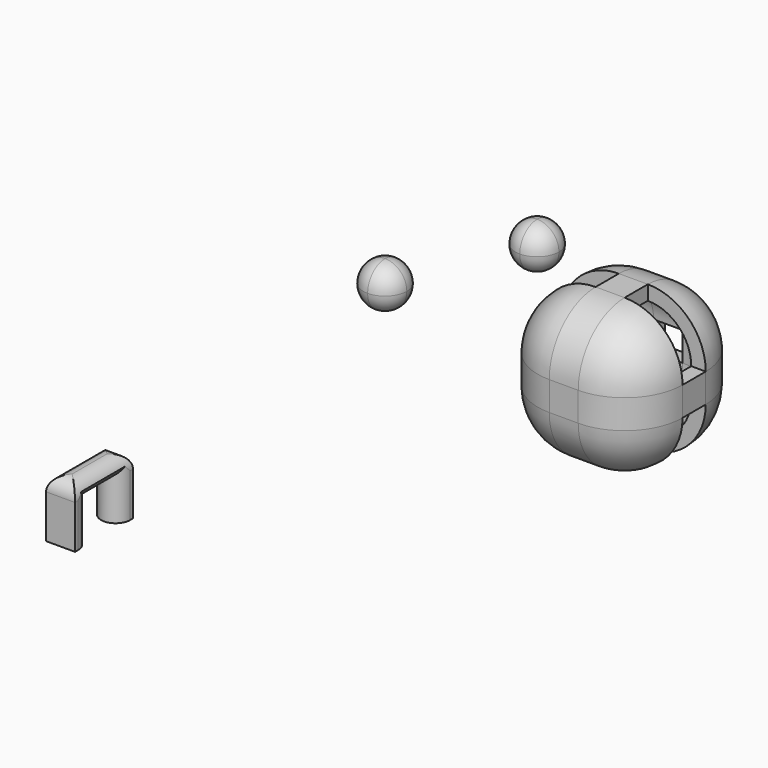
from build123d import *

# Parameters (mm, degrees)
F0_W         = 25.4
F0_H         = 25.4
F1_DEPTH     = 25.4
F2_R         = 10.16
F3_W         = 5.08
F3_H         = 12.7
F4_DEPTH     = 12.7
F6_DEPTH     = 5.08
F7_T1_DEPTH  = 5.08
F7_T3_DEPTH  = 6.35
F7_T5_DEPTH  = 9.525
F7_T7_DEPTH  = 12.7
F7_T13_DEPTH = 19.05
F7_T17_DEPTH = 11.43
F7_T24_DEPTH = 19.05
F7_T28_DEPTH = 11.43
F7_T35_DEPTH = 19.05
F7_T39_DEPTH = 11.43
F7_T46_DEPTH = 11.43
F7_T50_DEPTH = 19.05
F7_T57_DEPTH = 15.875
F7_T61_DEPTH = 12.7
F7_T68_DEPTH = 12.7
F7_T72_DEPTH = 15.875
F7_T79_DEPTH = 15.875
F7_T83_DEPTH = 12.7
F7_T90_DEPTH = 12.7
F7_T94_DEPTH = 15.875
F8_T         = 2.54
F9_W         = 7.62
F9_H         = 7.62
F10_DEPTH    = 7.62
F11_R        = 3.80999
F11_2_R      = 3.80999
F13_DEPTH    = 2.54
F15_DEPTH    = 2.54


# Not quite as in the source:
# - a fillet or chamfer that OpenCascade refuses, or shapes differently, is made with other operations: its cross-section is extruded or revolved along the edge and cut away or added
# - a fillet or chamfer is up to 0.001 mm smaller than in the source, because OpenCascade refuses the exact size
# - a shell that OpenCascade refuses in one call is made with other operations: the cavity is built on its own and cut out


with BuildPart() as f1:
    # F0 (on Top) → F1 (new body)
    with BuildSketch(Plane.XY):
        with Locations((-12.7, 12.7)):
            Rectangle(F0_W, F0_H)
    extrude(amount=F1_DEPTH)

    # F2
    f2_edges = [f1.edges().sort_by_distance(p)[0] for p in [
        (-12.7, 0, 25.4),
        (0, 12.7, 25.4),
        (-12.7, 25.4, 25.4),
        (-25.4, 12.7, 25.4),
        (-25.4, 0, 12.7),
        (0, 0, 12.7),
        (-12.7, 0, 0),
        (-25.4, 25.4, 12.7),
        (-25.4, 12.7, 0),
        (0, 25.4, 12.7),
        (-12.7, 25.4, 0),
        (0, 12.7, 0),
    ]]
    fillet(f2_edges, radius=F2_R)

    # F8: shell of thickness 2.54, made by hand


with BuildPart() as f4:
    # F3 (on Top) → F4 (new body)
    with BuildSketch(Plane.XY):
        with Locations((-51.7951508677, -55.0308073103)):
            Rectangle(F3_W, F3_H)
    extrude(amount=F4_DEPTH)

    # F5 (on face) → F6 (cut)
    with BuildSketch(Plane.YZ.offset(-49.2551508677)):
        Polygon((-58.2058073103, 0), (-55.0308073103, 0), (-51.8558073103, 0), (-51.8558073103, 9.525), (-58.2058073103, 9.525), align=None)
    extrude(amount=-F6_DEPTH, mode=Mode.SUBTRACT)

    # F7: fillet of radius 2.54 on 10 edges, made by hand

    # F7_s2 → F7_t1 (cut)
    with BuildSketch(Plane.YZ.offset(-54.3351508677)):
        with BuildLine():
            ThreePointArc((-51.2208073103, 12.7), (-49.4247560861, 11.9560512242), (-48.6808073103, 10.16))
            Line((-48.6808073103, 10.16), (-48.6300073103, 10.16))
            Line((-48.6300073103, 10.16), (-48.6300073103, 12.7508))
            Line((-48.6300073103, 12.7508), (-51.2208073103, 12.7508))
            Line((-51.2208073103, 12.7508), (-51.2208073103, 12.7))
        make_face()
        with BuildLine():
            ThreePointArc((-61.3808073103, 10.16), (-60.6368585346, 11.9560512242), (-58.8408073103, 12.7))
            Line((-58.8408073103, 12.7), (-58.8408073103, 12.7508))
            Line((-58.8408073103, 12.7508), (-61.4316073103, 12.7508))
            Line((-61.4316073103, 12.7508), (-61.4316073103, 10.16))
            Line((-61.4316073103, 10.16), (-61.3808073103, 10.16))
        make_face()
    extrude(amount=F7_T1_DEPTH, mode=Mode.SUBTRACT)

    # F7_s4 → F7_t3 (cut)
    with BuildSketch(Plane.XZ.offset(51.8558073103)):
        with BuildLine():
            ThreePointArc((-51.7951508677, 9.525), (-49.9990996435, 10.2689487758), (-49.2551508677, 12.065))
            Line((-49.2551508677, 12.065), (-49.2043508677, 12.065))
            Line((-49.2043508677, 12.065), (-49.2043508677, 9.4742))
            Line((-49.2043508677, 9.4742), (-51.7951508677, 9.4742))
            Line((-51.7951508677, 9.4742), (-51.7951508677, 9.525))
        make_face()
        with BuildLine():
            ThreePointArc((-54.3351508677, 12.065), (-53.5912020919, 10.2689487758), (-51.7951508677, 9.525))
            Line((-51.7951508677, 9.525), (-51.7951508677, 9.4742))
            Line((-51.7951508677, 9.4742), (-54.3859508677, 9.4742))
            Line((-54.3859508677, 9.4742), (-54.3859508677, 12.065))
            Line((-54.3859508677, 12.065), (-54.3351508677, 12.065))
        make_face()
    extrude(amount=F7_T3_DEPTH, mode=Mode.SUBTRACT)

    # F7_s6 → F7_t5 (cut)
    with BuildSketch(Plane.XY):
        with BuildLine():
            ThreePointArc((-51.7951508677, -58.2058073103), (-49.9990996435, -58.9497560861), (-49.2551508677, -60.7458073103))
            Line((-49.2551508677, -60.7458073103), (-49.2043508677, -60.7458073103))
            Line((-49.2043508677, -60.7458073103), (-49.2043508677, -58.1550073103))
            Line((-49.2043508677, -58.1550073103), (-51.7951508677, -58.1550073103))
            Line((-51.7951508677, -58.1550073103), (-51.7951508677, -58.2058073103))
        make_face()
        with BuildLine():
            ThreePointArc((-51.7951508677, -51.8558073103), (-49.9990996435, -51.1118585346), (-49.2551508677, -49.3158073103))
            Line((-49.2551508677, -49.3158073103), (-49.2043508677, -49.3158073103))
            Line((-49.2043508677, -49.3158073103), (-49.2043508677, -51.9066073103))
            Line((-49.2043508677, -51.9066073103), (-51.7951508677, -51.9066073103))
            Line((-51.7951508677, -51.9066073103), (-51.7951508677, -51.8558073103))
        make_face()
        with BuildLine():
            ThreePointArc((-54.3351508677, -49.3158073103), (-53.5912020919, -51.1118585346), (-51.7951508677, -51.8558073103))
            Line((-51.7951508677, -51.8558073103), (-51.7951508677, -51.9066073103))
            Line((-51.7951508677, -51.9066073103), (-54.3859508677, -51.9066073103))
            Line((-54.3859508677, -51.9066073103), (-54.3859508677, -49.3158073103))
            Line((-54.3859508677, -49.3158073103), (-54.3351508677, -49.3158073103))
        make_face()
        with BuildLine():
            ThreePointArc((-54.3351508677, -60.7458073103), (-53.5912020919, -58.9497560861), (-51.7951508677, -58.2058073103))
            Line((-51.7951508677, -58.2058073103), (-51.7951508677, -58.1550073103))
            Line((-51.7951508677, -58.1550073103), (-54.3859508677, -58.1550073103))
            Line((-54.3859508677, -58.1550073103), (-54.3859508677, -60.7458073103))
            Line((-54.3859508677, -60.7458073103), (-54.3351508677, -60.7458073103))
        make_face()
    extrude(amount=F7_T5_DEPTH, mode=Mode.SUBTRACT)

    # F7_s8 → F7_t7 (cut)
    with BuildSketch(Plane.XZ.offset(48.6808073103)):
        with BuildLine():
            ThreePointArc((-54.3351508677, 10.16), (-53.5912020919, 11.9560512242), (-51.7951508677, 12.7))
            Line((-51.7951508677, 12.7), (-51.7951508677, 12.7508))
            Line((-51.7951508677, 12.7508), (-54.3859508677, 12.7508))
            Line((-54.3859508677, 12.7508), (-54.3859508677, 10.16))
            Line((-54.3859508677, 10.16), (-54.3351508677, 10.16))
        make_face()
        with BuildLine():
            ThreePointArc((-51.7951508677, 12.7), (-49.9990996435, 11.9560512242), (-49.2551508677, 10.16))
            Line((-49.2551508677, 10.16), (-49.2043508677, 10.16))
            Line((-49.2043508677, 10.16), (-49.2043508677, 12.7508))
            Line((-49.2043508677, 12.7508), (-51.7951508677, 12.7508))
            Line((-51.7951508677, 12.7508), (-51.7951508677, 12.7))
        make_face()
    extrude(amount=F7_T7_DEPTH, mode=Mode.SUBTRACT)


with BuildPart() as f7_tool11:
    # F7_s12 → F7_t13 (new body)
    with BuildSketch(Plane.XZ.offset(61.3808073103)):
        with BuildLine():
            ThreePointArc((-51.7951508677, 12.7), (-49.9990996435, 11.9560512242), (-49.2551508677, 10.16))
            Line((-49.2551508677, 10.16), (-49.2043508677, 10.16))
            Line((-49.2043508677, 10.16), (-49.2043508677, 12.7508))
            Line((-49.2043508677, 12.7508), (-51.7951508677, 12.7508))
            Line((-51.7951508677, 12.7508), (-51.7951508677, 12.7))
        make_face()
    extrude(amount=-F7_T13_DEPTH)

    split(bisect_by=Plane.XZ.offset(48.6808073103), keep=Keep.BOTTOM)


with BuildPart() as f7_tool15:
    # F7_s16 → F7_t17 (new body)
    with BuildSketch(Plane.YZ.offset(-42.9051508677)):
        with BuildLine():
            ThreePointArc((-51.2208073103, 12.7), (-49.4247560861, 11.9560512242), (-48.6808073103, 10.16))
            Line((-48.6808073103, 10.16), (-48.6300073103, 10.16))
            Line((-48.6300073103, 10.16), (-48.6300073103, 12.7508))
            Line((-48.6300073103, 12.7508), (-51.2208073103, 12.7508))
            Line((-51.2208073103, 12.7508), (-51.2208073103, 12.7))
        make_face()
    extrude(amount=-F7_T17_DEPTH)

    split(bisect_by=Plane.YZ.offset(-49.2551508677), keep=Keep.TOP)


with BuildPart() as f7_tool11_1:
    add(f7_tool11.part)

    # F7_t19: intersect F7_tool15
    add(f7_tool15.part, mode=Mode.INTERSECT)


with BuildPart() as f4_1:
    add(f4.part)

    # F7_t9: cut F7_tool11
    add(f7_tool11_1.part, mode=Mode.SUBTRACT)


with BuildPart() as f7_tool22:
    # F7_s23 → F7_t24 (new body)
    with BuildSketch(Plane.XZ.offset(42.3308073103)):
        with BuildLine():
            ThreePointArc((-54.3351508677, 10.16), (-53.5912020919, 11.9560512242), (-51.7951508677, 12.7))
            Line((-51.7951508677, 12.7), (-51.7951508677, 12.7508))
            Line((-51.7951508677, 12.7508), (-54.3859508677, 12.7508))
            Line((-54.3859508677, 12.7508), (-54.3859508677, 10.16))
            Line((-54.3859508677, 10.16), (-54.3351508677, 10.16))
        make_face()
    extrude(amount=F7_T24_DEPTH)

    split(bisect_by=Plane.XZ.offset(48.6808073103), keep=Keep.BOTTOM)


with BuildPart() as f7_tool26:
    # F7_s27 → F7_t28 (new body)
    with BuildSketch(Plane.YZ.offset(-49.2551508677)):
        with BuildLine():
            ThreePointArc((-51.2208073103, 12.7), (-49.4247560861, 11.9560512242), (-48.6808073103, 10.16))
            Line((-48.6808073103, 10.16), (-48.6300073103, 10.16))
            Line((-48.6300073103, 10.16), (-48.6300073103, 12.7508))
            Line((-48.6300073103, 12.7508), (-51.2208073103, 12.7508))
            Line((-51.2208073103, 12.7508), (-51.2208073103, 12.7))
        make_face()
    extrude(amount=-F7_T28_DEPTH)

    split(bisect_by=Plane.YZ.offset(-54.3351508677), keep=Keep.BOTTOM)


with BuildPart() as f7_tool22_1:
    add(f7_tool22.part)

    # F7_t30: intersect F7_tool26
    add(f7_tool26.part, mode=Mode.INTERSECT)


with BuildPart() as f4_2:
    add(f4_1.part)

    # F7_t20: cut F7_tool22
    add(f7_tool22_1.part, mode=Mode.SUBTRACT)


with BuildPart() as f7_tool33:
    # F7_s34 → F7_t35 (new body)
    with BuildSketch(Plane.XZ.offset(48.6808073103)):
        with BuildLine():
            ThreePointArc((-54.3351508677, 10.16), (-53.5912020919, 11.9560512242), (-51.7951508677, 12.7))
            Line((-51.7951508677, 12.7), (-51.7951508677, 12.7508))
            Line((-51.7951508677, 12.7508), (-54.3859508677, 12.7508))
            Line((-54.3859508677, 12.7508), (-54.3859508677, 10.16))
            Line((-54.3859508677, 10.16), (-54.3351508677, 10.16))
        make_face()
    extrude(amount=F7_T35_DEPTH)

    split(bisect_by=Plane.XZ.offset(61.3808073103), keep=Keep.TOP)


with BuildPart() as f7_tool37:
    # F7_s38 → F7_t39 (new body)
    with BuildSketch(Plane.YZ.offset(-60.6851508677)):
        with BuildLine():
            ThreePointArc((-61.3808073103, 10.16), (-60.6368585346, 11.9560512242), (-58.8408073103, 12.7))
            Line((-58.8408073103, 12.7), (-58.8408073103, 12.7508))
            Line((-58.8408073103, 12.7508), (-61.4316073103, 12.7508))
            Line((-61.4316073103, 12.7508), (-61.4316073103, 10.16))
            Line((-61.4316073103, 10.16), (-61.3808073103, 10.16))
        make_face()
    extrude(amount=F7_T39_DEPTH)

    split(bisect_by=Plane.YZ.offset(-54.3351508677), keep=Keep.BOTTOM)


with BuildPart() as f7_tool33_1:
    add(f7_tool33.part)

    # F7_t41: intersect F7_tool37
    add(f7_tool37.part, mode=Mode.INTERSECT)


with BuildPart() as f4_3:
    add(f4_2.part)

    # F7_t31: cut F7_tool33
    add(f7_tool33_1.part, mode=Mode.SUBTRACT)


with BuildPart() as f7_tool44:
    # F7_s45 → F7_t46 (new body)
    with BuildSketch(Plane.YZ.offset(-54.3351508677)):
        with BuildLine():
            ThreePointArc((-61.3808073103, 10.16), (-60.6368585346, 11.9560512242), (-58.8408073103, 12.7))
            Line((-58.8408073103, 12.7), (-58.8408073103, 12.7508))
            Line((-58.8408073103, 12.7508), (-61.4316073103, 12.7508))
            Line((-61.4316073103, 12.7508), (-61.4316073103, 10.16))
            Line((-61.4316073103, 10.16), (-61.3808073103, 10.16))
        make_face()
    extrude(amount=F7_T46_DEPTH)

    split(bisect_by=Plane.YZ.offset(-49.2551508677), keep=Keep.TOP)


with BuildPart() as f7_tool48:
    # F7_s49 → F7_t50 (new body)
    with BuildSketch(Plane.XZ.offset(67.7308073103)):
        with BuildLine():
            ThreePointArc((-51.7951508677, 12.7), (-49.9990996435, 11.9560512242), (-49.2551508677, 10.16))
            Line((-49.2551508677, 10.16), (-49.2043508677, 10.16))
            Line((-49.2043508677, 10.16), (-49.2043508677, 12.7508))
            Line((-49.2043508677, 12.7508), (-51.7951508677, 12.7508))
            Line((-51.7951508677, 12.7508), (-51.7951508677, 12.7))
        make_face()
    extrude(amount=-F7_T50_DEPTH)

    split(bisect_by=Plane.XZ.offset(61.3808073103), keep=Keep.TOP)


with BuildPart() as f7_tool44_1:
    add(f7_tool44.part)

    # F7_t52: intersect F7_tool48
    add(f7_tool48.part, mode=Mode.INTERSECT)


with BuildPart() as f4_4:
    add(f4_3.part)

    # F7_t42: cut F7_tool44
    add(f7_tool44_1.part, mode=Mode.SUBTRACT)


with BuildPart() as f7_tool55:
    # F7_s56 → F7_t57 (new body)
    with BuildSketch(Plane.XY):
        with BuildLine():
            ThreePointArc((-51.7951508677, -51.8558073103), (-49.9990996435, -51.1118585346), (-49.2551508677, -49.3158073103))
            Line((-49.2551508677, -49.3158073103), (-49.2043508677, -49.3158073103))
            Line((-49.2043508677, -49.3158073103), (-49.2043508677, -51.9066073103))
            Line((-49.2043508677, -51.9066073103), (-51.7951508677, -51.9066073103))
            Line((-51.7951508677, -51.9066073103), (-51.7951508677, -51.8558073103))
        make_face()
    extrude(amount=F7_T57_DEPTH)

    split(bisect_by=Plane.XY.offset(9.525), keep=Keep.TOP)


with BuildPart() as f7_tool59:
    # F7_s60 → F7_t61 (new body)
    with BuildSketch(Plane.XZ.offset(45.5058073103)):
        with BuildLine():
            ThreePointArc((-51.7951508677, 9.525), (-49.9990996435, 10.2689487758), (-49.2551508677, 12.065))
            Line((-49.2551508677, 12.065), (-49.2043508677, 12.065))
            Line((-49.2043508677, 12.065), (-49.2043508677, 9.4742))
            Line((-49.2043508677, 9.4742), (-51.7951508677, 9.4742))
            Line((-51.7951508677, 9.4742), (-51.7951508677, 9.525))
        make_face()
    extrude(amount=F7_T61_DEPTH)

    split(bisect_by=Plane.XZ.offset(51.8558073103), keep=Keep.BOTTOM)


with BuildPart() as f7_tool55_1:
    add(f7_tool55.part)

    # F7_t63: intersect F7_tool59
    add(f7_tool59.part, mode=Mode.INTERSECT)


with BuildPart() as f4_5:
    add(f4_4.part)

    # F7_t53: cut F7_tool55
    add(f7_tool55_1.part, mode=Mode.SUBTRACT)


with BuildPart() as f7_tool66:
    # F7_s67 → F7_t68 (new body)
    with BuildSketch(Plane.XZ.offset(51.8558073103)):
        with BuildLine():
            ThreePointArc((-51.7951508677, 9.525), (-49.9990996435, 10.2689487758), (-49.2551508677, 12.065))
            Line((-49.2551508677, 12.065), (-49.2043508677, 12.065))
            Line((-49.2043508677, 12.065), (-49.2043508677, 9.4742))
            Line((-49.2043508677, 9.4742), (-51.7951508677, 9.4742))
            Line((-51.7951508677, 9.4742), (-51.7951508677, 9.525))
        make_face()
    extrude(amount=F7_T68_DEPTH)

    split(bisect_by=Plane.XZ.offset(58.2058073103), keep=Keep.TOP)


with BuildPart() as f7_tool70:
    # F7_s71 → F7_t72 (new body)
    with BuildSketch(Plane.XY.offset(15.875)):
        with BuildLine():
            ThreePointArc((-51.7951508677, -58.2058073103), (-49.9990996435, -58.9497560861), (-49.2551508677, -60.7458073103))
            Line((-49.2551508677, -60.7458073103), (-49.2043508677, -60.7458073103))
            Line((-49.2043508677, -60.7458073103), (-49.2043508677, -58.1550073103))
            Line((-49.2043508677, -58.1550073103), (-51.7951508677, -58.1550073103))
            Line((-51.7951508677, -58.1550073103), (-51.7951508677, -58.2058073103))
        make_face()
    extrude(amount=-F7_T72_DEPTH)

    split(bisect_by=Plane.XY.offset(9.525), keep=Keep.TOP)


with BuildPart() as f7_tool66_1:
    add(f7_tool66.part)

    # F7_t74: intersect F7_tool70
    add(f7_tool70.part, mode=Mode.INTERSECT)


with BuildPart() as f4_6:
    add(f4_5.part)

    # F7_t64: cut F7_tool66
    add(f7_tool66_1.part, mode=Mode.SUBTRACT)


with BuildPart() as f7_tool77:
    # F7_s78 → F7_t79 (new body)
    with BuildSketch(Plane.XY):
        with BuildLine():
            ThreePointArc((-54.3351508677, -49.3158073103), (-53.5912020919, -51.1118585346), (-51.7951508677, -51.8558073103))
            Line((-51.7951508677, -51.8558073103), (-51.7951508677, -51.9066073103))
            Line((-51.7951508677, -51.9066073103), (-54.3859508677, -51.9066073103))
            Line((-54.3859508677, -51.9066073103), (-54.3859508677, -49.3158073103))
            Line((-54.3859508677, -49.3158073103), (-54.3351508677, -49.3158073103))
        make_face()
    extrude(amount=F7_T79_DEPTH)

    split(bisect_by=Plane.XY.offset(9.525), keep=Keep.TOP)


with BuildPart() as f7_tool81:
    # F7_s82 → F7_t83 (new body)
    with BuildSketch(Plane.XZ.offset(45.5058073103)):
        with BuildLine():
            ThreePointArc((-54.3351508677, 12.065), (-53.5912020919, 10.2689487758), (-51.7951508677, 9.525))
            Line((-51.7951508677, 9.525), (-51.7951508677, 9.4742))
            Line((-51.7951508677, 9.4742), (-54.3859508677, 9.4742))
            Line((-54.3859508677, 9.4742), (-54.3859508677, 12.065))
            Line((-54.3859508677, 12.065), (-54.3351508677, 12.065))
        make_face()
    extrude(amount=F7_T83_DEPTH)

    split(bisect_by=Plane.XZ.offset(51.8558073103), keep=Keep.BOTTOM)


with BuildPart() as f7_tool77_1:
    add(f7_tool77.part)

    # F7_t85: intersect F7_tool81
    add(f7_tool81.part, mode=Mode.INTERSECT)


with BuildPart() as f4_7:
    add(f4_6.part)

    # F7_t75: cut F7_tool77
    add(f7_tool77_1.part, mode=Mode.SUBTRACT)


with BuildPart() as f7_tool88:
    # F7_s89 → F7_t90 (new body)
    with BuildSketch(Plane.XZ.offset(51.8558073103)):
        with BuildLine():
            ThreePointArc((-54.3351508677, 12.065), (-53.5912020919, 10.2689487758), (-51.7951508677, 9.525))
            Line((-51.7951508677, 9.525), (-51.7951508677, 9.4742))
            Line((-51.7951508677, 9.4742), (-54.3859508677, 9.4742))
            Line((-54.3859508677, 9.4742), (-54.3859508677, 12.065))
            Line((-54.3859508677, 12.065), (-54.3351508677, 12.065))
        make_face()
    extrude(amount=F7_T90_DEPTH)

    split(bisect_by=Plane.XZ.offset(58.2058073103), keep=Keep.TOP)


with BuildPart() as f7_tool92:
    # F7_s93 → F7_t94 (new body)
    with BuildSketch(Plane.XY.offset(15.875)):
        with BuildLine():
            ThreePointArc((-54.3351508677, -60.7458073103), (-53.5912020919, -58.9497560861), (-51.7951508677, -58.2058073103))
            Line((-51.7951508677, -58.2058073103), (-51.7951508677, -58.1550073103))
            Line((-51.7951508677, -58.1550073103), (-54.3859508677, -58.1550073103))
            Line((-54.3859508677, -58.1550073103), (-54.3859508677, -60.7458073103))
            Line((-54.3859508677, -60.7458073103), (-54.3351508677, -60.7458073103))
        make_face()
    extrude(amount=-F7_T94_DEPTH)

    split(bisect_by=Plane.XY.offset(9.525), keep=Keep.TOP)


with BuildPart() as f7_tool88_1:
    add(f7_tool88.part)

    # F7_t96: intersect F7_tool92
    add(f7_tool92.part, mode=Mode.INTERSECT)


with BuildPart() as f4_8:
    add(f4_7.part)

    # F7_t86: cut F7_tool88
    add(f7_tool88_1.part, mode=Mode.SUBTRACT)

    # F12 (on face) → F13 (cut)
    with BuildSketch(Plane(origin=(0, 0, 0), x_dir=(1, 0, 0), z_dir=(0, 0, -1))):
        with BuildLine():
            ThreePointArc((-54.3351508677, 60.7458073103), (-53.5912020919, 58.9497560861), (-51.7951508677, 58.2058073103))
            ThreePointArc((-51.7951508677, 58.2058073103), (-49.9990996435, 58.9497560861), (-49.2551508677, 60.7458073103))
            Line((-49.2551508677, 60.7458073103), (-49.2551508677, 61.3808073103))
            Line((-49.2551508677, 61.3808073103), (-54.3351508677, 61.3808073103))
            Line((-54.3351508677, 61.3808073103), (-54.3351508677, 60.7458073103))
        make_face()
    extrude(amount=-F13_DEPTH, mode=Mode.SUBTRACT)

    # F14 (on face) → F15 (cut)
    with BuildSketch(Plane(origin=(0, 0, 0), x_dir=(1, 0, 0), z_dir=(0, 0, -1))):
        with BuildLine():
            Line((-54.3351508677, 48.6808073103), (-49.2551508677, 48.6808073103))
            Line((-49.2551508677, 48.6808073103), (-49.2551508677, 49.3158073103))
            ThreePointArc((-49.2551508677, 49.3158073103), (-49.9990996435, 51.1118585346), (-51.7951508677, 51.8558073103))
            ThreePointArc((-51.7951508677, 51.8558073103), (-53.591202092, 51.1118585346), (-54.3351508677, 49.3158073103))
            Line((-54.3351508677, 49.3158073103), (-54.3351508677, 48.6808073103))
        make_face()
    extrude(amount=-F15_DEPTH, mode=Mode.SUBTRACT)


with BuildPart() as f8_core1:
    # F8_t2: copy of F1
    add(f1.part)

    # the walls: a layer under each face that stays
    f8_faces = [f8_core1.faces().sort_by_distance(p)[0] for p in [
        (-12.7, 0, 12.7),
        (-12.7, 2.9757951031, 22.4242048969),
        (-22.4242048969, 2.9757951031, 12.7),
        (-2.9757951031, 2.9757951031, 12.7),
        (-12.7, 2.9757951031, 2.9757951031),
        (-22.4242048969, 5.08, 20.32),
        (-2.9757951031, 5.08, 20.32),
        (-12.7, 12.7, 25.4),
        (-20.32, 5.08, 2.9757951031),
        (-25.4, 12.7, 12.7),
        (-5.08, 5.08, 2.9757951031),
        (0, 12.7, 12.7),
        (-12.7, 12.7, 0),
        (-12.7, 22.4242048969, 22.4242048969),
        (-22.4242048969, 22.4242048969, 12.7),
        (-2.9757951031, 22.4242048969, 12.7),
        (-12.7, 22.4242048969, 2.9757951031),
        (-22.4242048969, 20.32, 20.32),
        (-5.08, 22.4242048969, 20.32),
        (-20.32, 20.32, 2.9757951031),
        (-5.08, 20.32, 2.9757951031),
    ]]
    thicken(f8_faces, amount=-F8_T, mode=Mode.SUBTRACT)


with BuildPart() as f1_1:
    add(f1.part)

    # what is left inside the walls is the cavity
    f8_cavity = [f8_core1.part.solids().sort_by_distance(p)[0] for p in [
        (-17.925097, 7.474903, 3.582883),
    ]]
    add(f8_cavity, mode=Mode.SUBTRACT)


with BuildPart() as f10:
    # F9 (on Top) → F10 (new body)
    with BuildSketch(Plane.XY):
        with Locations((-64.336842434, 25.3919505193)):
            Rectangle(F9_W, F9_H)
    extrude(amount=F10_DEPTH)

    # F11#2 (radius 3.81 in the source; OpenCascade refuses exactly that, so slightly less here)
    f11_2_edges = [f10.edges().sort_by_distance(p)[0] for p in [
        (-64.336842, 29.201951, 0),
        (-68.146842, 25.391951, 0),
        (-64.336842, 21.581951, 0),
        (-60.526842, 25.391951, 0),
        (-60.526842, 29.201951, 3.81),
        (-68.146842, 29.201951, 3.81),
        (-64.336842, 29.201951, 7.62),
        (-68.146842, 21.581951, 3.81),
        (-68.146842, 25.391951, 7.62),
        (-64.336842, 21.581951, 7.62),
        (-60.526842, 25.391951, 7.62),
        (-60.526842, 21.581951, 3.81),
    ]]
    fillet(f11_2_edges, radius=F11_2_R)


with BuildPart() as f10b:
    # F9 (on Top) → F10, piece 2 (new body)
    with BuildSketch(Plane.XY):
        with Locations((-55.3688526402, 47.5126730917)):
            Rectangle(F9_W, F9_H)
    extrude(amount=F10_DEPTH)

    # F11 (radius 3.81 in the source; OpenCascade refuses exactly that, so slightly less here)
    f11_edges = [f10b.edges().sort_by_distance(p)[0] for p in [
        (-51.558853, 43.702673, 3.81),
        (-51.558853, 51.322673, 3.81),
        (-51.558853, 47.512673, 0),
        (-51.558853, 47.512673, 7.62),
        (-59.178853, 51.322673, 3.81),
        (-55.368853, 51.322673, 0),
        (-55.368853, 51.322673, 7.62),
        (-59.178853, 43.702673, 3.81),
        (-59.178853, 47.512673, 0),
        (-59.178853, 47.512673, 7.62),
        (-55.368853, 43.702673, 0),
        (-55.368853, 43.702673, 7.62),
    ]]
    fillet(f11_edges, radius=F11_R)


solid = Compound([f4_8.part, f1_1.part, f10.part, f10b.part])
